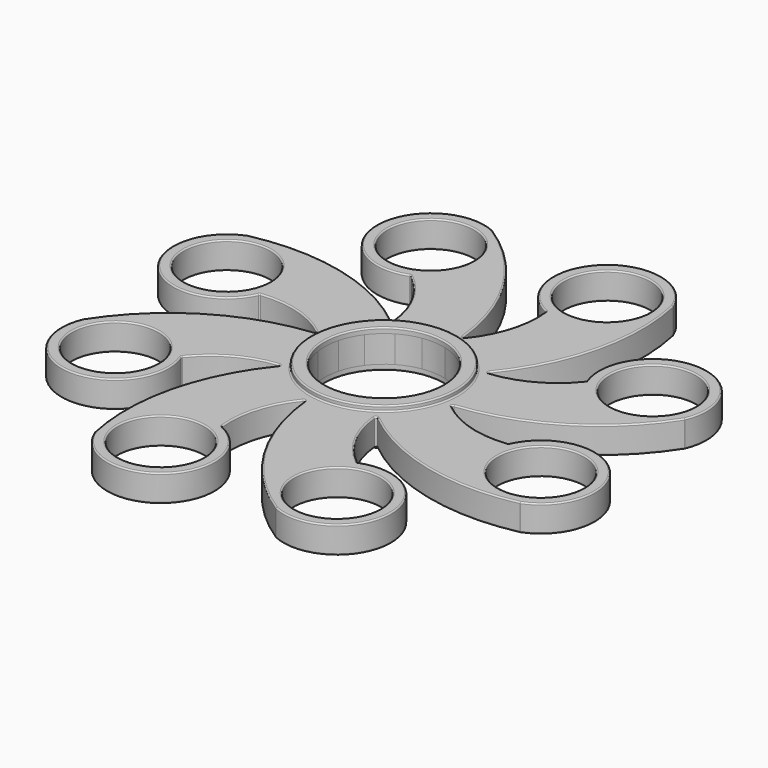
from build123d import *
from build123d import SkipClean  # not in build123d's __all__

# Parameters (mm, degrees)
F0_R     = 8
F1_DEPTH = 5
F2_R     = 13.5
F2_R_2   = 11
F3_DEPTH = 1
F4_R     = 13.5
F4_R_2   = 11
F5_DEPTH = 1
F6_F1_R  = 0.25
F6_F2_R  = 0.25
F6_F3_R  = 0.2499


# Not quite as in the source:
# - a fillet or chamfer is up to 0.001 mm smaller than in the source, because OpenCascade refuses the exact size


with BuildPart() as f1:
    # F0 (on Top) → F1 (new body)
    with BuildSketch(Plane.XY):
        with BuildLine():
            ThreePointArc((12.1448214975, 8.3589112783), (20.0933463392, 23.9727429948), (20.3385560646, 41.4916088319))
            ThreePointArc((20.3385560646, 41.4916088319), (4.0757669045, 45.0747374034), (7.0581741801, 28.691136808))
            ThreePointArc((7.0581741801, 28.691136808), (6.3752082202, 21.1293566354), (2.677042789, 14.4983284855))
            ThreePointArc((2.677042789, 14.4983284855), (-2.743147682, 31.1594305884), (-14.9574670545, 43.7205288802))
            ThreePointArc((-14.9574670545, 43.7205288802), (-28.9906500615, 34.7546548949), (-15.2968145713, 25.2785802225))
            ThreePointArc((-15.2968145713, 25.2785802225), (-10.432758395, 19.448664323), (-8.3589112783, 12.1448214975))
            ThreePointArc((-8.3589112783, 12.1448214975), (-23.9727429948, 20.0933463392), (-41.4916088319, 20.3385560646))
            ThreePointArc((-41.4916088319, 20.3385560646), (-45.0747374034, 4.0757669045), (-28.691136808, 7.0581741801))
            ThreePointArc((-28.691136808, 7.0581741801), (-21.1293566354, 6.3752082202), (-14.4983284855, 2.677042789))
            ThreePointArc((-14.4983284855, 2.677042789), (-31.1594305884, -2.743147682), (-43.7205288802, -14.9574670545))
            ThreePointArc((-43.7205288802, -14.9574670545), (-34.7546548949, -28.9906500615), (-25.2785802225, -15.2968145713))
            ThreePointArc((-25.2785802225, -15.2968145713), (-19.448664323, -10.432758395), (-12.1448214975, -8.3589112783))
            ThreePointArc((-12.1448214975, -8.3589112783), (-20.0933463392, -23.9727429948), (-20.3385560646, -41.4916088319))
            ThreePointArc((-20.3385560646, -41.4916088319), (-4.0757669045, -45.0747374034), (-7.0581741801, -28.691136808))
            ThreePointArc((-7.0581741801, -28.691136808), (-6.3752082202, -21.1293566354), (-2.677042789, -14.4983284855))
            ThreePointArc((-2.677042789, -14.4983284855), (2.743147682, -31.1594305884), (14.9574670545, -43.7205288802))
            ThreePointArc((14.9574670545, -43.7205288802), (28.9906500615, -34.7546548949), (15.2968145713, -25.2785802225))
            ThreePointArc((15.2968145713, -25.2785802225), (10.432758395, -19.448664323), (8.3589112783, -12.1448214975))
            ThreePointArc((8.3589112783, -12.1448214975), (23.9727429948, -20.0933463392), (41.4916088319, -20.3385560646))
            ThreePointArc((41.4916088319, -20.3385560646), (45.0747374034, -4.0757669045), (28.691136808, -7.0581741801))
            ThreePointArc((28.691136808, -7.0581741801), (21.1293566354, -6.3752082202), (14.4983284855, -2.677042789))
            ThreePointArc((14.4983284855, -2.677042789), (31.1594305884, 2.743147682), (43.7205288802, 14.9574670545))
            ThreePointArc((43.7205288802, 14.9574670545), (34.7546548949, 28.9906500615), (25.2785802225, 15.2968145713))
            ThreePointArc((25.2785802225, 15.2968145713), (19.448664323, 10.432758395), (12.1448214975, 8.3589112783))
        make_face()
        with Locations((-11.0155462887, -37.8747747579)):
            Circle(F0_R, mode=Mode.SUBTRACT)
        with Locations((-34.5706775464, -18.992342588)):
            Circle(F0_R, mode=Mode.SUBTRACT)
        with Locations((18.992342588, -34.5706775464)):
            Circle(F0_R, mode=Mode.SUBTRACT)
        with Locations((37.8747747579, -11.0155462887)):
            Circle(F0_R, mode=Mode.SUBTRACT)
        with Locations((-37.8747747579, 11.0155462887)):
            Circle(F0_R, mode=Mode.SUBTRACT)
        with Locations((-18.992342588, 34.5706775464)):
            Circle(F0_R, mode=Mode.SUBTRACT)
        with BuildLine():
            ThreePointArc((-5.5273043451, 9.5104630106), (-3.6488460909, 10.3771827682), (-1.641326988, 10.8768582651))
            ThreePointArc((-1.641326988, 10.8768582651), (0.6000816993, 10.9836197109), (2.8165185029, 10.6333072711))
            ThreePointArc((2.8165185029, 10.6333072711), (8.1909138184, 7.3422701407), (10.8768582651, 1.641326988))
            ThreePointArc((10.8768582651, 1.641326988), (10.9691713661, 0.8229699521), (11, 0))
            ThreePointArc((11, 0), (10.9079416019, -1.4201443619), (10.6333072711, -2.8165185029))
            ThreePointArc((10.6333072711, -2.8165185029), (9.9179001194, -4.7576524906), (8.8516936806, -6.5305067939))
            ThreePointArc((8.8516936806, -6.5305067939), (7.3422701407, -8.1909138184), (5.5273043451, -9.5104630106))
            ThreePointArc((5.5273043451, -9.5104630106), (3.6488460909, -10.3771827682), (1.641326988, -10.8768582651))
            ThreePointArc((1.641326988, -10.8768582651), (-0.6000816993, -10.9836197109), (-2.8165185029, -10.6333072711))
            ThreePointArc((-2.8165185029, -10.6333072711), (-4.7576524906, -9.9179001194), (-6.5305067939, -8.8516936806))
            ThreePointArc((-6.5305067939, -8.8516936806), (-8.1909138184, -7.3422701407), (-9.5104630106, -5.5273043451))
            ThreePointArc((-9.5104630106, -5.5273043451), (-10.3771827682, -3.6488460909), (-10.8768582651, -1.641326988))
            ThreePointArc((-10.8768582651, -1.641326988), (-10.9836197109, 0.6000816993), (-10.6333072711, 2.8165185029))
            ThreePointArc((-10.6333072711, 2.8165185029), (-9.9179001194, 4.7576524906), (-8.8516936806, 6.5305067939))
            ThreePointArc((-8.8516936806, 6.5305067939), (-7.3422701407, 8.1909138184), (-5.5273043451, 9.5104630106))
        make_face(mode=Mode.SUBTRACT)
        with Locations((34.5706775464, 18.992342588)):
            Circle(F0_R, mode=Mode.SUBTRACT)
        with Locations((11.0155462887, 37.8747747579)):
            Circle(F0_R, mode=Mode.SUBTRACT)
    extrude(amount=F1_DEPTH)

    # F2 (on face) → F3 (join)
    with BuildSketch(Plane.XY.offset(5)):
        Circle(F2_R)
        Circle(F2_R_2, mode=Mode.SUBTRACT)
    with SkipClean():  # cleaning this boolean's faces spoils the solid; the shape is the same uncleaned
        extrude(amount=F3_DEPTH)

    # F4 (on face) → F5 (join)
    with BuildSketch(Plane(origin=(0, 0, 0), x_dir=(1, 0, 0), z_dir=(0, 0, -1))):
        Circle(F4_R)
        Circle(F4_R_2, mode=Mode.SUBTRACT)
    with SkipClean():  # cleaning this boolean's faces spoils the solid; the shape is the same uncleaned
        extrude(amount=F5_DEPTH)

    # F6: fillet of radius 0.25 on 111 edges, made by hand

    # F6_f1
    f6_f1_edges = [f1.edges().sort_by_distance(p)[0] for p in [
        (25.2785802225, 15.2968145713, 2.5),
        (-25.2785802225, -15.2968145713, 2.5),
        (12.1448214975, 8.3589112783, 2.5),
        (8.3589112783, -12.1448214975, 2.5),
        (15.2968145713, -25.2785802225, 2.5),
        (-13.5, 0, 5),
        (14.4983284855, -2.677042789, 2.5),
        (-14.4983284855, 2.677042789, 2.5),
        (-15.2968145713, 25.2785802225, 2.5),
        (28.691136808, -7.0581741801, 2.5),
        (-2.677042789, -14.4983284855, 2.5),
        (-7.0581741801, -28.691136808, 2.5),
        (7.0581741801, 28.691136808, 2.5),
        (-28.691136808, 7.0581741801, 2.5),
        (-12.1448214975, -8.3589112783, 2.5),
        (2.677042789, 14.4983284855, 2.5),
        (-13.5, 0, 0),
        (-8.3589112783, 12.1448214975, 2.5),
    ]]
    fillet(f6_f1_edges, radius=F6_F1_R)

    # F6_f2
    f6_f2_edges = [f1.edges().sort_by_distance(p)[0] for p in [
        (43.7205288802, 14.9574670545, 2.5),
        (-42.5706775464, -18.992342588, 5),
        (-43.7205288802, -14.9574670545, 2.5),
        (20.3385560646, 41.4916088319, 2.5),
        (-19.0155462887, -37.8747747579, 0),
        (-19.0155462887, -37.8747747579, 5),
        (-13.5, 0, 6),
        (41.4916088319, -20.3385560646, 2.5),
        (14.9574670545, -43.7205288802, 2.5),
        (-42.5706775464, -18.992342588, 0),
        (10.992342588, -34.5706775464, 5),
        (29.8747747579, -11.0155462887, 5),
        (-45.8747747579, 11.0155462887, 5),
        (-26.992342588, 34.5706775464, 5),
        (26.5706775464, 18.992342588, 5),
        (3.0155462887, 37.8747747579, 5),
        (-11, 0, 6),
        (29.8747747579, -11.0155462887, 0),
        (-14.9574670545, 43.7205288802, 2.5),
        (-20.3385560646, -41.4916088319, 2.5),
        (10.992342588, -34.5706775464, 0),
        (-41.4916088319, 20.3385560646, 2.5),
        (-45.8747747579, 11.0155462887, 0),
        (26.5706775464, 18.992342588, 0),
        (-26.992342588, 34.5706775464, 0),
        (3.0155462887, 37.8747747579, 0),
        (-11, 0, -1),
        (-13.5, 0, -1),
    ]]
    fillet(f6_f2_edges, radius=F6_F2_R)

    # F6_f3 (radius 0.25 in the source; OpenCascade refuses exactly that, so slightly less here)
    f6_f3_edges = [f1.edges().sort_by_distance(p)[0] for p in [
        (34.8155049486, 28.9893451159, 0),
        (34.8155049486, 28.9893451159, 5),
        (45.1168421532, -4.119717126, 5),
        (-34.8155049486, -28.9893451159, 5),
        (-6.4409274381, -21.3470545458, 5),
        (-19.6490704964, -10.5402235591, 5),
        (-28.9893451159, 34.8155049486, 5),
        (-31.4043562382, -2.8921921614, 5),
        (-34.8155049486, -28.9893451159, 0),
        (10.5402235591, -19.6490704964, 5),
        (20.161144565, 24.2513219447, 0),
        (20.161144565, 24.2513219447, 5),
        (24.2513219447, -20.161144565, 0),
        (24.2513219447, -20.161144565, 5),
        (28.9893451159, -34.8155049486, 0),
        (28.9893451159, -34.8155049486, 5),
        (31.4043562382, 2.8921921614, 0),
        (31.4043562382, 2.8921921614, 5),
        (-21.3470545458, 6.4409274381, 5),
        (-45.1168421532, 4.119717126, 5),
        (-24.2513219447, 20.161144565, 5),
        (-10.5402235591, 19.6490704964, 5),
        (-20.161144565, -24.2513219447, 5),
        (-2.8921921614, 31.4043562382, 5),
        (-4.119717126, -45.1168421532, 5),
        (6.4409274381, 21.3470545458, 5),
        (4.119717126, 45.1168421532, 5),
        (2.8921921614, -31.4043562382, 5),
        (19.6490704964, 10.5402235591, 5),
        (21.3470545458, -6.4409274381, 5),
        (-31.4043562382, -2.8921921614, 0),
        (-28.9893451159, 34.8155049486, 0),
        (45.1168421532, -4.119717126, 0),
        (2.8921921614, -31.4043562382, 0),
        (-4.119717126, -45.1168421532, 0),
        (4.119717126, 45.1168421532, 0),
        (-45.1168421532, 4.119717126, 0),
        (-20.161144565, -24.2513219447, 0),
        (-2.8921921614, 31.4043562382, 0),
        (-21.3470545458, 6.4409274381, 0),
        (6.4409274381, 21.3470545458, 0),
        (19.6490704964, 10.5402235591, 0),
        (-24.2513219447, 20.161144565, 0),
        (-10.5402235591, 19.6490704964, 0),
        (-19.6490704964, -10.5402235591, 0),
        (-6.4409274381, -21.3470545458, 0),
        (10.5402235591, -19.6490704964, 0),
        (21.3470545458, -6.4409274381, 0),
        (28.6673358228, -7.028258003, 0),
        (14.8747407825, -2.7982850369, 0),
        (15.301138665, -25.2405964527, 0),
        (8.5393437504, -12.496716401, 0),
        (-7.028258003, -28.6673358228, 0),
        (-2.7982850369, -14.8747407825, 0),
        (-25.2405964527, -15.301138665, 0),
        (-12.496716401, -8.5393437504, 0),
        (-15.3011386647, 25.2405964526, 0),
        (-8.5393437504, 12.496716401, 0),
        (-41.4914757129, 20.3377909235, 0),
        (25.2405964526, 15.3011386647, 0),
        (12.496716401, 8.5393437504, 0),
        (7.0282580031, 28.6673358225, 0),
        (2.7982850369, 14.8747407825, 0),
        (-28.6673358225, 7.0282580031, 0),
        (-14.8747407825, 2.7982850369, 0),
        (-14.9579139617, 43.7198937144, 0),
        (-20.3377909235, -41.4914757129, 0),
        (20.3377909235, 41.4914757129, 0),
        (14.9579139617, -43.7198937144, 0),
        (41.4914757129, -20.3377909235, 0),
        (-43.7198937144, -14.9579139617, 0),
        (28.6673358228, -7.028258003, 5),
        (14.8747407825, -2.7982850369, 5),
        (25.2405964526, 15.3011386647, 5),
        (12.496716401, 8.5393437504, 5),
        (-2.7982850369, -14.8747407825, 5),
        (14.9579139617, -43.7198937144, 5),
        (20.3377909235, 41.4914757129, 5),
        (7.0282580031, 28.6673358225, 5),
        (2.7982850369, 14.8747407825, 5),
        (-20.3377909235, -41.4914757129, 5),
        (-7.028258003, -28.6673358228, 5),
        (-14.9579139617, 43.7198937144, 5),
        (-12.496716401, -8.5393437504, 5),
        (-15.3011386647, 25.2405964526, 5),
        (-8.5393437504, 12.496716401, 5),
        (-41.4914757129, 20.3377909235, 5),
        (-28.6673358225, 7.0282580031, 5),
        (-14.8747407825, 2.7982850369, 5),
        (43.7198937144, 14.9579139617, 5),
        (43.7198937144, 14.9579139617, 0),
        (15.301138665, -25.2405964527, 5),
        (8.5393437504, -12.496716401, 5),
        (41.4914757129, -20.3377909235, 5),
        (-43.7198937144, -14.9579139617, 5),
        (-25.2405964527, -15.301138665, 5),
    ]]
    fillet(f6_f3_edges, radius=F6_F3_R)


solid = f1.part
